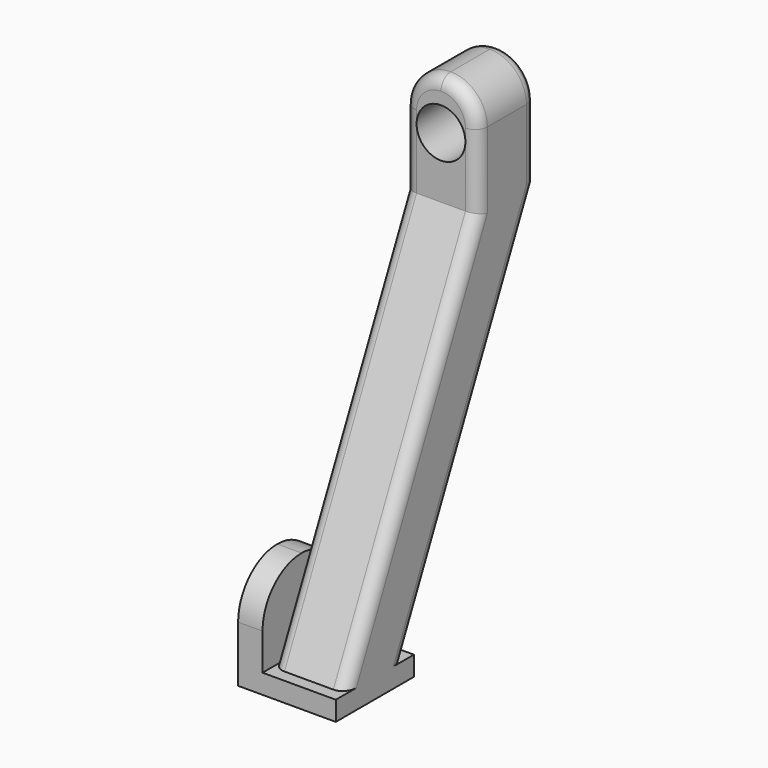
from build123d import *

# Parameters (mm, degrees)
F0_W      = 4
F0_H      = 4
F1_DEPTH  = 0.8
F4_DEPTH  = 1.5
F5_R      = 1
F6_DEPTH  = 10.2624610432
F7_R      = 1.49999
F8_R      = 0.49999
F10_DEPTH = 1


# Not quite as in the source:
# - a fillet or chamfer is up to 0.001 mm smaller than in the source, because OpenCascade refuses the exact size


with BuildPart() as f1:
    # F0 (on Top) → F1 (new body)
    with BuildSketch(Plane.XY):
        with Locations((2, 2)):
            Rectangle(F0_W, F0_H)
    extrude(amount=F1_DEPTH)

    # F3 (on offset) → F4 (join, symmetric)
    with BuildSketch(Plane.YZ.offset(2.5)):
        Polygon((0.5, 0.8), (3.5, 0.8), (10.2614610432, 15.3), (10.2614610432, 19.8), (7.2614610432, 19.8), (7.2614610432, 15.3), align=None)
    extrude(amount=F4_DEPTH, both=True)

    # F5 (on face) → F6 (cut, through all)
    with BuildSketch(Plane(origin=(0, 10.2614610432, 0), x_dir=(-1, 0, 0), z_dir=(0, 1, 0))):
        with Locations((-2.5, 17.8)):
            Circle(F5_R)
    extrude(amount=-F6_DEPTH, mode=Mode.SUBTRACT)

    # F7 (radius 1.5 in the source; OpenCascade refuses exactly that, so slightly less here)
    f7_edges = [f1.edges().sort_by_distance(p)[0] for p in [
        (1, 8.761461, 19.8),
        (4, 8.761461, 19.8),
    ]]
    fillet(f7_edges, radius=F7_R)

    # F8 (radius 0.5 in the source; OpenCascade refuses exactly that, so slightly less here)
    f8_edges = [f1.edges().sort_by_distance(p)[0] for p in [
        (1, 6.880731, 8.05),
        (1, 10.261461, 16.800005),
        (3.560663, 10.261461, 19.360663),
        (4, 6.880731, 8.05),
        (1, 3.880731, 8.05),
        (1, 7.261461, 16.800005),
        (4, 3.880731, 8.05),
    ]]
    fillet(f8_edges, radius=F8_R)

    # F9 (on face) → F10 (join)
    with BuildSketch(Plane(origin=(0, 0, 0), x_dir=(0, -1, 0), z_dir=(-1, 0, 0))):
        with BuildLine():
            Line((-4, 2.3), (-4, 0.8))
            Line((-4, 0.8), (0, 0.8))
            Line((0, 0.8), (0, 2.3))
            ThreePointArc((0, 2.3), (-0.5857864376, 3.7142135624), (-2, 4.3))
            ThreePointArc((-2, 4.3), (-3.4142135624, 3.7142135624), (-4, 2.3))
        make_face()
    extrude(amount=-F10_DEPTH)


solid = f1.part
